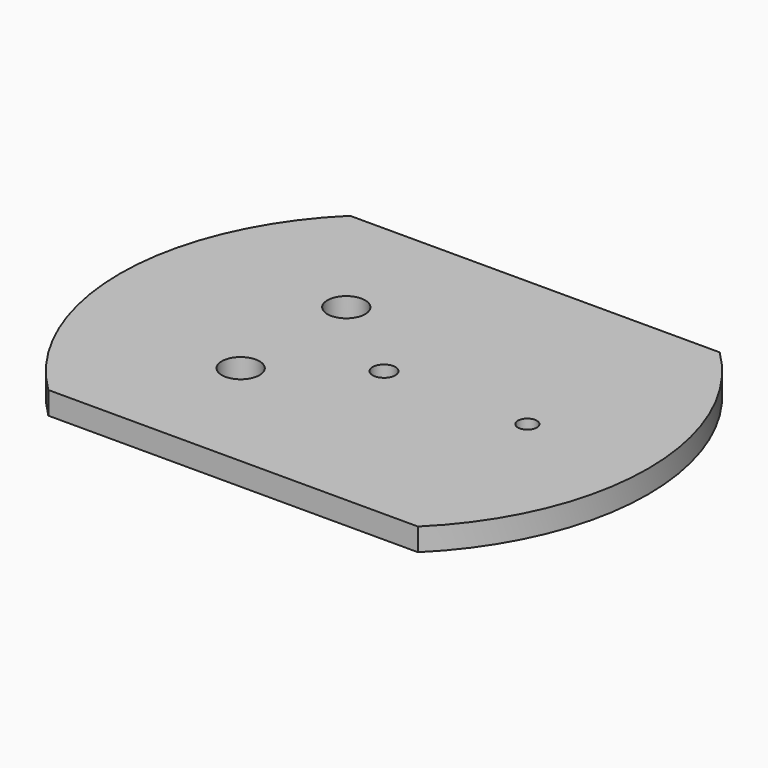
from build123d import *

# Parameters (mm, degrees)
F0_R     = 35
F1_DEPTH = 3
F2_R     = 5
F3_DEPTH = 5
F4_R     = 1.5
F4_R_2   = 2.5
F4_R_3   = 1.25
F5_DEPTH = 8.001
F6_W     = 70
F6_H     = 50
F7_DEPTH = 10


# Not quite as in the source:
# - a feature names something its author has since deleted; it is built from what else it names


with BuildPart() as f1:
    # F0 (on Top) → F1 (new body)
    with BuildSketch(Plane.XY):
        Circle(F0_R)
    extrude(amount=F1_DEPTH)

    # F2 (on face) → F3 (join)
    with BuildSketch(Plane(origin=(0, 0, 0), x_dir=(1, 0, 0), z_dir=(0, 0, -1))):
        Circle(F2_R)
    extrude(amount=F3_DEPTH)

    # F4 (on face) → F5 (cut, through all)
    with BuildSketch(Plane.XY.offset(3)):
        Circle(F4_R)
        with Locations((-12, 8.75)):
            Circle(F4_R_2)
        with Locations((-12, -8.75)):
            Circle(F4_R_2)
        with Locations((19, 0)):
            Circle(F4_R_3)
    extrude(amount=-F5_DEPTH, mode=Mode.SUBTRACT)

    # F6 (on Top) → F7 (intersect, symmetric)
    with BuildSketch(Plane.XY):
        Rectangle(F6_W, F6_H)
    extrude(amount=F7_DEPTH, both=True, mode=Mode.INTERSECT)


solid = f1.part
